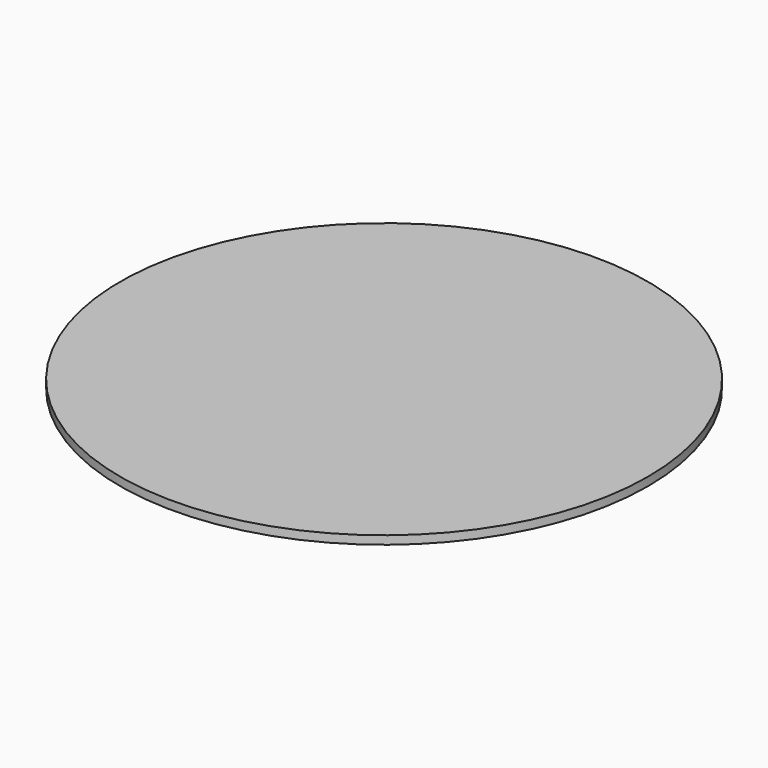
from build123d import *

# Parameters (mm, degrees)
F6_R     = 78.5901187679
F7_DEPTH = 2.5


# Not quite as in the source:
# - a feature of the source that left no trace in its solid (it failed there, or was rolled back) is left out
# - the program builds the solid bodies; features that only make, move or delete a surface that nothing else refers to are left out


with BuildPart() as f7:
    # F6 (on offset) → F7 (new body)
    with BuildSketch(Plane.XY.offset(-47)):
        Circle(F6_R)
    extrude(amount=F7_DEPTH)


solid = f7.part
